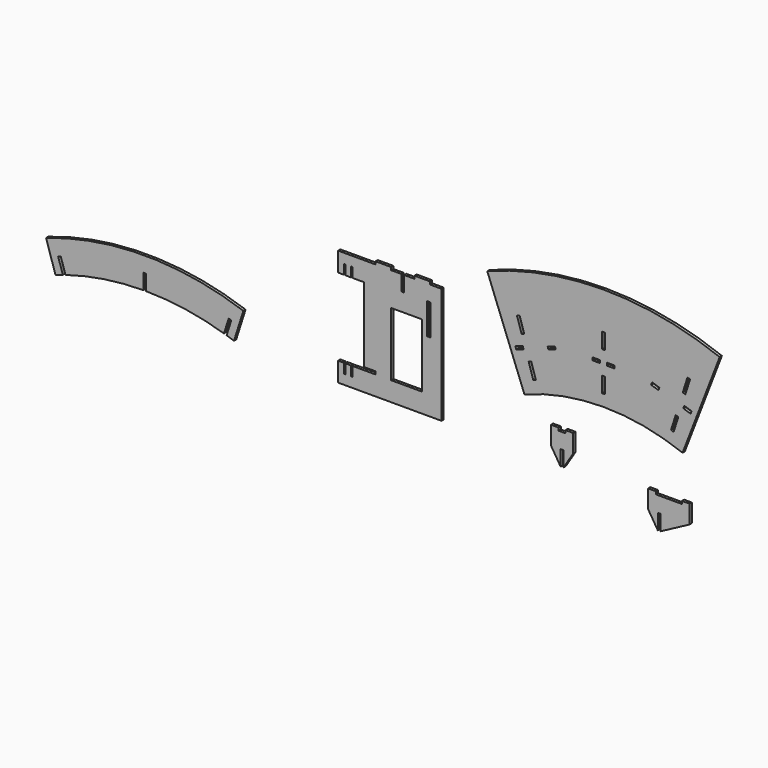
from build123d import *

# Parameters (mm, degrees)
F0_W     = 24.7396
F0_H     = 203.2
F0_W_2   = 101.6
F0_H_2   = 18.1428571429
F1_DEPTH = 18.1356
F0_W_3   = 50.8
F0_W_4   = 18.1428571429
F0_H_3   = 101.6


# Not quite as in the source:
# - a feature names something its author has since deleted; it is built from what else it names


with BuildPart() as f1:
    # F0 (on Front) → F1 (new body)
    with BuildSketch(Plane.XZ):
        Polygon((-1433.7949680964, -199.4009857178), (-1509.9949680964, -199.4009857178), (-1679.3283014297, -199.4009857178), (-1679.3283014297, -326.4009857178), (-1641.2283014297, -326.4009857178), (-1641.2283014297, -262.9009857178), (-1632.3383014297, -262.9009857178), (-1632.3383014297, -326.4009857178), (-1594.2383014297, -326.4009857178), (-1594.2383014297, -262.9009857178), (-1585.3483014297, -262.9009857178), (-1585.3483014297, -326.4009857178), (-1509.9949680964, -326.4009857178), (-1509.9949680964, -815.8589857178), (-1433.7949680964, -815.8589857178), (-1433.7949680964, -834.4009857178), (-1509.9949680964, -834.4009857178), (-1585.3483014297, -834.4009857178), (-1585.3483014297, -897.9009857178), (-1594.2383014297, -897.9009857178), (-1594.2383014297, -834.4009857178), (-1632.3383014297, -834.4009857178), (-1632.3383014297, -897.9009857178), (-1641.2283014297, -897.9009857178), (-1641.2283014297, -834.4009857178), (-1679.3283014297, -834.4009857178), (-1679.3283014297, -961.4009857178), (-1509.9949680964, -961.4009857178), (-1001.9949680964, -961.4009857178), (-1001.9949680964, -199.4009857178), (-1078.1949680964, -199.4009857178), (-1179.7949680964, -199.4009857178), (-1246.923539525, -199.4009857178), (-1246.923539525, -301.0009857178), (-1265.0663966678, -301.0009857178), (-1265.0663966678, -199.4009857178), (-1332.1949680964, -199.4009857178), align=None)
        Polygon((-1332.1949680964, -815.8589857178), (-1332.1949680964, -417.1152714321), (-1128.9949680964, -417.1152714321), (-1128.9949680964, -834.4009857178), (-1332.1949680964, -834.4009857178), align=None, mode=Mode.SUBTRACT)
        with Locations((-1085.5244682964, -402.6009857178)):
            Rectangle(F0_W, F0_H, mode=Mode.SUBTRACT)
        with Locations((-1382.9949680964, -190.3295571463)):
            Rectangle(F0_W_2, F0_H_2)
        with Locations((-1128.9949680964, -190.3295571463)):
            Rectangle(F0_W_2, F0_H_2)
    extrude(amount=F1_DEPTH)


with BuildPart() as f1b:
    # F0 (on Front) → F1, piece 2 (new body)
    with BuildSketch(Plane.XZ):
        Polygon((-233.0102896554, -768.8084903581), (-283.8102896554, -768.8084903581), (-283.8102896554, -870.4084903581), (-220.3102896554, -972.0084903581), (-220.3102896554, -870.4084903581), (-202.1674325126, -870.4084903581), (-202.1674325126, -972.0084903581), (-138.6674325126, -870.4084903581), (-138.6674325126, -768.8084903581), (-189.4674325126, -768.8084903581), align=None)
        with Locations((-164.0674325126, -759.7370617867)):
            Rectangle(F0_W_3, F0_H_2)
        with Locations((-258.4102896554, -759.7370617867)):
            Rectangle(F0_W_3, F0_H_2)
    extrude(amount=F1_DEPTH)


with BuildPart() as f1c:
    # F0 (on Front) → F1, piece 3 (new body)
    with BuildSketch(Plane.XZ):
        with BuildLine():
            Line((579.0676760834, -631.9954848741), (822.7111688002, 0))
            ThreePointArc((822.7111688002, 0), (60.7111688002, 141.7950471023), (-701.2888311998, 0))
            Line((-701.2888311998, 0), (-457.6453384831, -631.9954848741))
            ThreePointArc((-457.6453384831, -631.9954848741), (60.7111688002, -535.538286231), (579.0676760834, -631.9954848741))
        make_face()
        Polygon((-399.240059352, -530.7352252685), (-430.0400839584, -433.9162266978), (-412.7509770708, -428.4162223038), (-381.9509524643, -525.2352208745), align=None, mode=Mode.SUBTRACT)
        Polygon((-511.2292535639, -389.3006605456), (-516.7292579579, -372.011553658), (-468.3197586725, -356.6115413548), (-462.8197542785, -373.9006482424), align=None, mode=Mode.SUBTRACT)
        Polygon((-458.9510139804, -283.1877244477), (-476.2401208681, -288.6877288417), (-507.0401454745, -191.8687302709), (-489.7510385869, -186.3687258769), align=None, mode=Mode.SUBTRACT)
        with Locations((60.7111688002, -408.5602558806)):
            Rectangle(F0_W_4, F0_H_3, mode=Mode.SUBTRACT)
        Polygon((534.1733146711, -428.4162223038), (551.4624215588, -433.9162266978), (520.6623969523, -530.7352252685), (503.3732900647, -525.2352208745), align=None, mode=Mode.SUBTRACT)
        Polygon((589.7420962729, -356.6115413548), (638.1515955583, -372.011553658), (632.6515911643, -389.3006605456), (584.2420918789, -373.9006482424), align=None, mode=Mode.SUBTRACT)
        Polygon((-300.3021495348, -322.2006069388), (-305.8021539288, -304.9115000511), (-257.3926546434, -289.5114877479), (-251.8926502494, -306.8005946355), align=None, mode=Mode.SUBTRACT)
        with Locations((13.5397402287, -281.5602558806)):
            Rectangle(F0_W_3, F0_H_2, mode=Mode.SUBTRACT)
        with Locations((107.8825973716, -281.5602558806)):
            Rectangle(F0_W_3, F0_H_2, mode=Mode.SUBTRACT)
        Polygon((373.3149878497, -306.8005946355), (378.8149922437, -289.5114877479), (427.2244915291, -304.9115000511), (421.7244871351, -322.2006069388), align=None, mode=Mode.SUBTRACT)
        Polygon((628.4624830749, -191.8687302709), (597.6624584684, -288.6877288417), (580.3733515808, -283.1877244477), (611.1733761872, -186.3687258769), align=None, mode=Mode.SUBTRACT)
        with Locations((60.7111688002, -154.5602558806)):
            Rectangle(F0_W_4, F0_H_3, mode=Mode.SUBTRACT)
    extrude(amount=F1_DEPTH)


with BuildPart() as f1d:
    # F0 (on Front) → F1, piece 4 (new body)
    with BuildSketch(Plane.XZ):
        with Locations((378.5851431642, -919.9377022879)):
            Rectangle(F0_W_3, F0_H_2)
        Polygon((403.9851431642, -929.0091308594), (353.1851431642, -929.0091308594), (353.1851431642, -1030.6091308594), (416.6851431642, -1132.2091308594), (416.6851431642, -1030.6091308594), (434.8280003071, -1030.6091308594), (434.8280003071, -1132.2091308594), (625.3280003071, -1030.6091308594), (625.3280003071, -929.0091308594), (574.5280003071, -929.0091308594), align=None)
        with Locations((599.9280003071, -919.9377022879)):
            Rectangle(F0_W_3, F0_H_2)
    extrude(amount=F1_DEPTH)


with BuildPart() as f1e:
    # F0 (on Front) → F1, piece 5 (new body)
    with BuildSketch(Plane.XZ):
        with BuildLine():
            Line((-2956.4141467797, -741.3827241583), (-2938.2712896368, -741.3827241583))
            Line((-2938.2712896368, -741.3827241583), (-2938.2712896368, -842.9827241583))
            Line((-2938.2712896368, -842.9827241583), (-2938.5207805782, -842.9827241583))
            ThreePointArc((-2938.5207805782, -842.9827241583), (-2680.2581818501, -863.2133164178), (-2427.7087045022, -920.8987414075))
            Line((-2427.7087045022, -920.8987414075), (-2427.6805354276, -920.8101927253))
            Line((-2427.6805354276, -920.8101927253), (-2396.8805108212, -823.9911941546))
            Line((-2396.8805108212, -823.9911941546), (-2379.5914039336, -829.4911985486))
            Line((-2379.5914039336, -829.4911985486), (-2410.39142854, -926.3101971193))
            ThreePointArc((-2410.39142854, -926.3101971193), (-2386.2394133775, -934.184590775), (-2362.202814439, -942.4045556973))
            Line((-2362.202814439, -942.4045556973), (-2361.9819292546, -941.7102094226))
            Line((-2361.9819292546, -941.7102094226), (-2331.1819046482, -844.8912108518))
            Line((-2331.1819046482, -844.8912108518), (-2300.5800248164, -748.6950747267))
            ThreePointArc((-2300.5800248164, -748.6950747267), (-2947.3427182083, -639.7607545087), (-3594.1054116001, -748.6950747267))
            Line((-3594.1054116001, -748.6950747267), (-3532.4826219776, -942.4045556973))
            ThreePointArc((-3532.4826219776, -942.4045556973), (-3508.446023039, -934.184590775), (-3484.2940078765, -926.3101971193))
            Line((-3484.2940078765, -926.3101971193), (-3515.0940324829, -829.4911985486))
            Line((-3515.0940324829, -829.4911985486), (-3497.8049255953, -823.9911941546))
            Line((-3497.8049255953, -823.9911941546), (-3467.0049009889, -920.8101927253))
            Line((-3467.0049009889, -920.8101927253), (-3466.9767319143, -920.8987414075))
            ThreePointArc((-3466.9767319143, -920.8987414075), (-3214.4272545664, -863.2133164178), (-2956.1646558383, -842.9827241583))
            Line((-2956.1646558383, -842.9827241583), (-2956.4141467797, -842.9827241583))
            Line((-2956.4141467797, -842.9827241583), (-2956.4141467797, -741.3827241583))
        make_face()
    extrude(amount=F1_DEPTH)


solid = Compound([f1.part, f1b.part, f1c.part, f1d.part, f1e.part])
